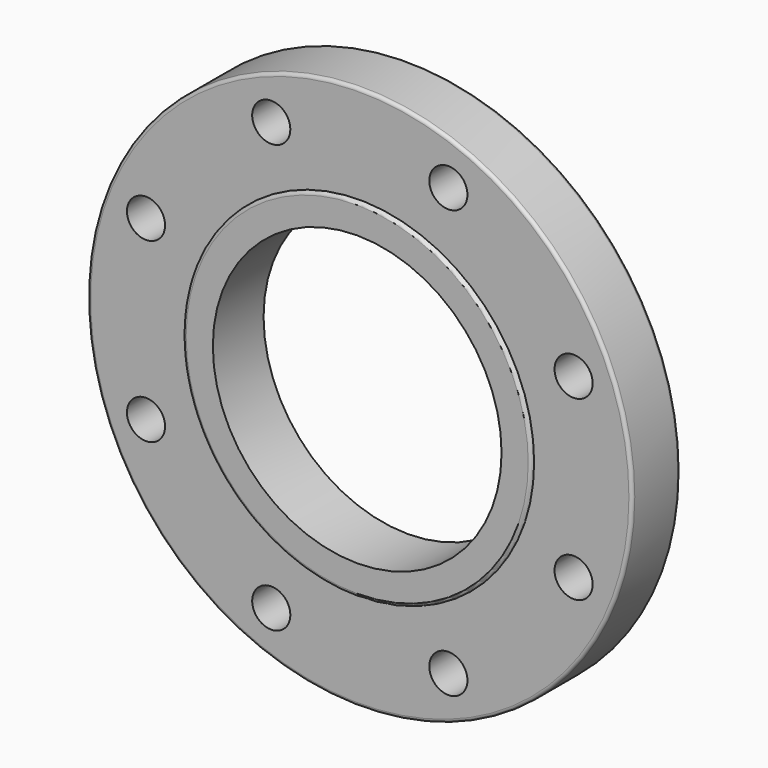
from build123d import *

# Parameters (mm, degrees)
F0_R     = 158.75
F0_R_2   = 11.1125
F0_R_3   = 84.1375
F1_DEPTH = 35.052
F2_R     = 101.6
F2_R_2   = 84.1375
F3_DEPTH = 1.905
F4_R     = 1.90499


# Not quite as in the source:
# - a fillet or chamfer is up to 0.001 mm smaller than in the source, because OpenCascade refuses the exact size


with BuildPart() as f1:
    # F0 (on Front) → F1 (new body)
    with BuildSketch(Plane.XZ):
        Circle(F0_R)
        with Locations((-51.6140452568, -124.6073280679)):
            Circle(F0_R_2, mode=Mode.SUBTRACT)
        with Locations((-124.6073280679, -51.6140452568)):
            Circle(F0_R_2, mode=Mode.SUBTRACT)
        with Locations((51.6140452568, -124.6073280679)):
            Circle(F0_R_2, mode=Mode.SUBTRACT)
        with Locations((124.6073280679, -51.6140452568)):
            Circle(F0_R_2, mode=Mode.SUBTRACT)
        with Locations((-124.6073280679, 51.6140452568)):
            Circle(F0_R_2, mode=Mode.SUBTRACT)
        with Locations((-51.6140452568, 124.6073280679)):
            Circle(F0_R_2, mode=Mode.SUBTRACT)
        Circle(F0_R_3, mode=Mode.SUBTRACT)
        with Locations((124.6073280679, 51.6140452568)):
            Circle(F0_R_2, mode=Mode.SUBTRACT)
        with Locations((51.6140452568, 124.6073280679)):
            Circle(F0_R_2, mode=Mode.SUBTRACT)
    extrude(amount=F1_DEPTH)

    # F2 (on face) → F3 (join)
    with BuildSketch(Plane.XZ.offset(35.052)):
        Circle(F2_R)
        Circle(F2_R_2, mode=Mode.SUBTRACT)
    extrude(amount=F3_DEPTH)

    # F4 (radius 1.905 in the source; OpenCascade refuses exactly that, so slightly less here)
    f4_edges = [f1.edges().sort_by_distance(p)[0] for p in [
        (-158.75, -35.052, 0),
        (-158.75, 0, 0),
        (-101.6, -36.957, 0),
    ]]
    fillet(f4_edges, radius=F4_R)


solid = f1.part
